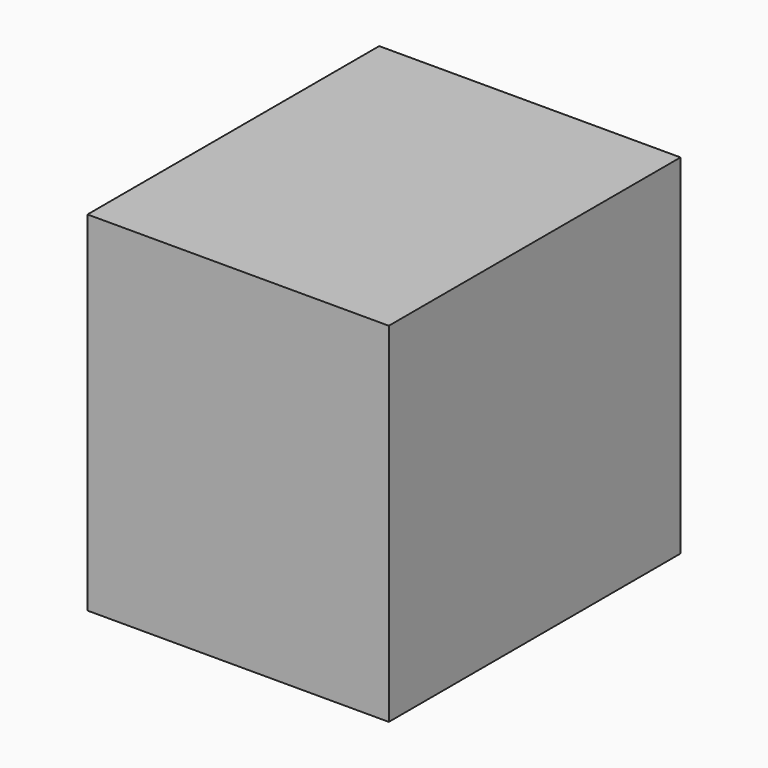
from build123d import *

# Parameters (mm, degrees)
F0_W     = 62.9755333066
F0_H     = 72.8878080845
F1_DEPTH = 76.2


# Not quite as in the source:
# - the program builds the solid bodies; features that only make, move or delete a surface that nothing else refers to are left out


with BuildPart() as f1:
    # F0 (on Front) → F1 (new body)
    with BuildSketch(Plane.XZ):
        with Locations((-122.280176729, 36.4439040422)):
            Rectangle(F0_W, F0_H)
    extrude(amount=F1_DEPTH)


solid = f1.part
